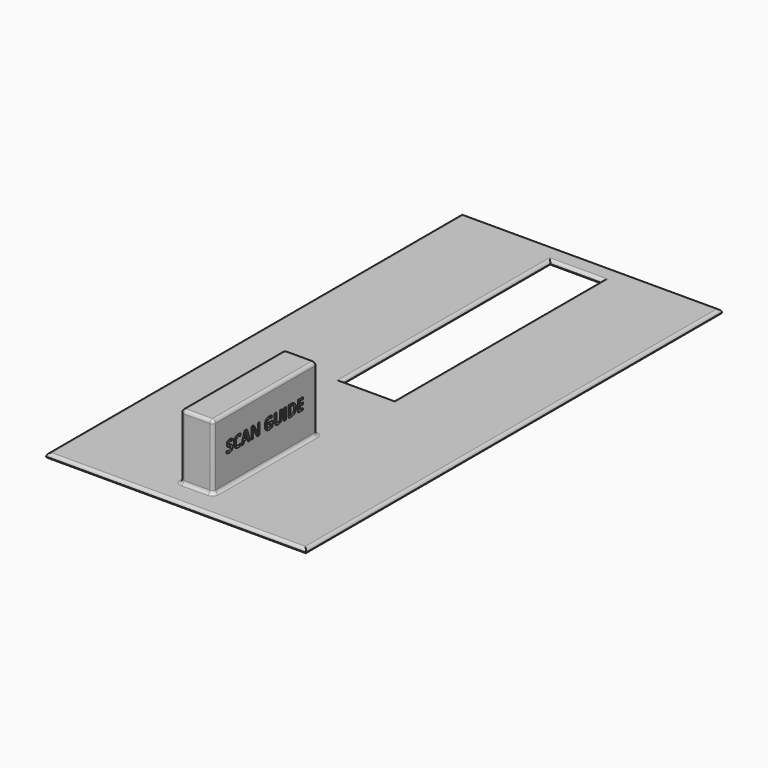
from build123d import *

# Parameters (mm, degrees)
F0_W          = 50.8
F0_H          = 101.5999981404
F1_DEPTH      = 1.016
F3_DEPTH      = 1.016
F4_DEPTH      = 12.7
F5_TEXT_SIZE  = 3.1394360757
F6_DEPTH      = 0.508
F7_TEXT_SIZE  = 2.617994417
F8_DEPTH      = 0.508
F9_R          = 0.635
F10_R         = 0.635
F11_T1_DEPTH  = 104.5099337067
F11_T3_DEPTH  = 53.7099355663
F11_T5_DEPTH  = 10.16
F11_T7_DEPTH  = 50.8
F11_T13_DEPTH = 11.6149677831
F11_T17_DEPTH = 52.2549677831
F11_T24_DEPTH = 52.2549677831
F11_T28_DEPTH = 11.6149677831
F11_T35_DEPTH = 52.2549677831
F11_T39_DEPTH = 11.6149677831
F11_T46_DEPTH = 11.6149677831
F11_T50_DEPTH = 52.2549677831


# Not quite as in the source:
# - a fillet or chamfer that OpenCascade refuses, or shapes differently, is made with other operations: its cross-section is extruded or revolved along the edge and cut away or added
# - Text() gives the source's letters only with a copy of the font that has no kerning and outlines rounded to 1/6400 em; it was checked with that copy


with BuildPart() as f1:
    # F0 (on Top) → F1 (new body)
    with BuildSketch(Plane.XY):
        with Locations((9.1255651787, -9.784890828)):
            Rectangle(F0_W, F0_H)
    extrude(amount=F1_DEPTH)

    # F2 (on face) → F3 (cut)
    with BuildSketch(Plane.XY.offset(1.016)):
        Polygon((4.0455651787, -13.5948917578), (9.1255651787, -13.5948917578), (14.2055651787, -13.5948917578), (14.2055651787, 37.2051082422), (9.1255651787, 37.2051082422), (4.0455651787, 37.2051082422), align=None)
    extrude(amount=-F3_DEPTH, mode=Mode.SUBTRACT)

    # F2 (on face) → F4 (join)
    with BuildSketch(Plane.XY.offset(1.016)):
        Polygon((12.3005651787, -30.1048898982), (9.1255651787, -30.1048898982), (5.9505651787, -30.1048898982), (5.9505651787, -55.5048898982), (9.1255651787, -55.5048898982), (12.3005651787, -55.5048898982), align=None)
    extrude(amount=F4_DEPTH)

    # F5 (on face) → F6 (cut)
    with BuildSketch(Plane.YZ.offset(12.3005651787)):
        with Locations((-52.3298898982, 6.7086623347)):
            Text('SCAN GUIDE', F5_TEXT_SIZE, font='Open Sans', font_style=FontStyle.BOLD, text_align=(TextAlign.LEFT, TextAlign.BOTTOM))
    extrude(amount=-F6_DEPTH, mode=Mode.SUBTRACT)

    # F7 (on face) → F8 (cut)
    with BuildSketch(Plane(origin=(5.9505651787, 0, 0), x_dir=(0, -1, 0), z_dir=(-1, 0, 0))):
        with Locations((33.1365615274, 6.3851709486)):
            Text('Physio Controls', F7_TEXT_SIZE, font='Open Sans', text_align=(TextAlign.LEFT, TextAlign.BOTTOM))
    extrude(amount=-F8_DEPTH, mode=Mode.SUBTRACT)

    # F9
    f9_edges = [f1.edges().sort_by_distance(p)[0] for p in [
        (12.300565, -42.80489, 1.016),
        (9.125565, -30.10489, 1.016),
        (5.950565, -42.80489, 1.016),
        (9.125565, -55.50489, 1.016),
        (9.125565, -30.10489, 13.716),
        (5.950565, -42.80489, 13.716),
        (9.125565, -55.50489, 13.716),
        (12.300565, -42.80489, 13.716),
        (5.950565, -55.50489, 7.366),
        (12.300565, -55.50489, 7.366),
        (12.300565, -30.10489, 7.366),
        (5.950565, -30.10489, 7.366),
    ]]
    fillet(f9_edges, radius=F9_R)

    # F10
    f10_edges = [f1.edges().sort_by_distance(p)[0] for p in [
        (12.935565, -42.80489, 1.016),
        (12.563591, -55.767916, 1.016),
        (12.563591, -29.841864, 1.016),
        (9.125565, -56.13989, 1.016),
        (9.125565, -29.46989, 1.016),
        (5.68754, -55.767916, 1.016),
        (5.68754, -29.841864, 1.016),
        (5.315565, -42.80489, 1.016),
        (34.525565, -9.784891, 1.016),
        (9.125565, -60.58489, 1.016),
        (9.125565, 41.015108, 1.016),
        (-16.274435, -9.784891, 1.016),
        (14.205565, 11.805108, 1.016),
        (9.125565, -13.594892, 1.016),
        (9.125565, 37.205108, 1.016),
        (4.045565, 11.805108, 1.016),
    ]]
    fillet(f10_edges, radius=F10_R)

    # F11: fillet of radius 0.635 on 8 edges, made by hand

    # F11_s2 → F11_t1 (cut)
    with BuildSketch(Plane.XZ.offset(-42.4700760253)):
        with BuildLine():
            ThreePointArc((34.5255651787, 0.381), (34.2913818894, 0.1037208832), (33.9435780654, 0))
            Line((33.9435780654, 0), (33.9435780654, -0.0127))
            Line((33.9435780654, -0.0127), (34.5255651787, -0.0127))
            Line((34.5255651787, -0.0127), (34.5382651787, 0))
            ThreePointArc((34.5382651787, 0), (34.5382651787, 0.1905), (34.537204921, 0.37592))
            Line((34.537204921, 0.37592), (34.5255651787, 0.381))
        make_face()
        with BuildLine():
            ThreePointArc((-16.2744348213, 0.381), (-16.0402515321, 0.1037208832), (-15.692447708, 0))
            Line((-15.692447708, 0), (-15.692447708, -0.0127))
            Line((-15.692447708, -0.0127), (-16.2744348213, -0.0127))
            Line((-16.2744348213, -0.0127), (-16.2871348213, 0))
            ThreePointArc((-16.2871348213, 0), (-16.2871348213, 0.1905), (-16.2860745636, 0.37592))
            Line((-16.2860745636, 0.37592), (-16.2744348213, 0.381))
        make_face()
    extrude(amount=F11_T1_DEPTH, mode=Mode.SUBTRACT)

    # F11_s4 → F11_t3 (cut)
    with BuildSketch(Plane.YZ.offset(-17.7294026045)):
        with BuildLine():
            ThreePointArc((-60.5848898982, 0.381), (-60.3507066089, 0.1037208832), (-60.0029027849, 0))
            Line((-60.0029027849, 0), (-60.0029027849, -0.0127))
            Line((-60.0029027849, -0.0127), (-60.5848898982, -0.0127))
            Line((-60.5848898982, -0.0127), (-60.5975898982, 0))
            ThreePointArc((-60.5975898982, 0), (-60.5975898982, 0.1905), (-60.5965296404, 0.37592))
            Line((-60.5965296404, 0.37592), (-60.5848898982, 0.381))
        make_face()
        with BuildLine():
            ThreePointArc((41.0151082422, 0.381), (40.7809249529, 0.1037208832), (40.4331211289, 0))
            Line((40.4331211289, 0), (40.4331211289, -0.0127))
            Line((40.4331211289, -0.0127), (41.0151082422, -0.0127))
            Line((41.0151082422, -0.0127), (41.0278082422, 0))
            ThreePointArc((41.0278082422, 0), (41.0278082422, 0.1905), (41.0267479844, 0.37592))
            Line((41.0267479844, 0.37592), (41.0151082422, 0.381))
        make_face()
    extrude(amount=F11_T3_DEPTH, mode=Mode.SUBTRACT)

    # F11_s6 → F11_t5 (cut)
    with BuildSketch(Plane.YZ.offset(4.0455651787)):
        with BuildLine():
            ThreePointArc((-13.5948917578, 0.381), (-13.8290750471, 0.1037208832), (-14.1768788711, 0))
            Line((-14.1768788711, 0), (-14.1768788711, -0.0127))
            Line((-14.1768788711, -0.0127), (-13.5948917578, -0.0127))
            Line((-13.5948917578, -0.0127), (-13.5821917578, 0))
            ThreePointArc((-13.5821917578, 0), (-13.5821917578, 0.1905), (-13.5832520156, 0.37592))
            Line((-13.5832520156, 0.37592), (-13.5948917578, 0.381))
        make_face()
        with BuildLine():
            ThreePointArc((37.2051082422, 0.381), (37.4392915314, 0.1037208832), (37.7870953554, 0))
            Line((37.7870953554, 0), (37.7870953554, -0.0127))
            Line((37.7870953554, -0.0127), (37.2051082422, -0.0127))
            Line((37.2051082422, -0.0127), (37.1924082422, 0))
            ThreePointArc((37.1924082422, 0), (37.1924082422, 0.1905), (37.1934684999, 0.37592))
            Line((37.1934684999, 0.37592), (37.2051082422, 0.381))
        make_face()
    extrude(amount=F11_T5_DEPTH, mode=Mode.SUBTRACT)

    # F11_s8 → F11_t7 (cut)
    with BuildSketch(Plane.XZ.offset(-37.2051082422)):
        with BuildLine():
            ThreePointArc((14.2055651787, 0.381), (14.4397484679, 0.1037208832), (14.787552292, 0))
            Line((14.787552292, 0), (14.787552292, -0.0127))
            Line((14.787552292, -0.0127), (14.2055651787, -0.0127))
            Line((14.2055651787, -0.0127), (14.1928651787, 0))
            ThreePointArc((14.1928651787, 0), (14.1928651787, 0.1905), (14.1939254364, 0.37592))
            Line((14.1939254364, 0.37592), (14.2055651787, 0.381))
        make_face()
        with BuildLine():
            ThreePointArc((4.0455651787, 0.381), (3.8113818894, 0.1037208832), (3.4635780654, 0))
            Line((3.4635780654, 0), (3.4635780654, -0.0127))
            Line((3.4635780654, -0.0127), (4.0455651787, -0.0127))
            Line((4.0455651787, -0.0127), (4.0582651787, 0))
            ThreePointArc((4.0582651787, 0), (4.0582651787, 0.1905), (4.057204921, 0.37592))
            Line((4.057204921, 0.37592), (4.0455651787, 0.381))
        make_face()
    extrude(amount=F11_T7_DEPTH, mode=Mode.SUBTRACT)


with BuildPart() as f11_tool11:
    # F11_s12 → F11_t13 (new body)
    with BuildSketch(Plane.YZ.offset(2.5905973955)):
        with BuildLine():
            ThreePointArc((-13.5948917578, 0.381), (-13.8290750471, 0.1037208832), (-14.1768788711, 0))
            Line((-14.1768788711, 0), (-14.1768788711, -0.0127))
            Line((-14.1768788711, -0.0127), (-13.5948917578, -0.0127))
            Line((-13.5948917578, -0.0127), (-13.5821917578, 0))
            ThreePointArc((-13.5821917578, 0), (-13.5821917578, 0.1905), (-13.5832520156, 0.37592))
            Line((-13.5832520156, 0.37592), (-13.5948917578, 0.381))
        make_face()
    extrude(amount=F11_T13_DEPTH)

    split(bisect_by=Plane.YZ.offset(4.0455651787), keep=Keep.BOTTOM)


with BuildPart() as f11_tool15:
    # F11_s16 → F11_t17 (new body)
    with BuildSketch(Plane.XZ.offset(-37.2051082422)):
        with BuildLine():
            ThreePointArc((4.0455651787, 0.381), (3.8113818894, 0.1037208832), (3.4635780654, 0))
            Line((3.4635780654, 0), (3.4635780654, -0.0127))
            Line((3.4635780654, -0.0127), (4.0455651787, -0.0127))
            Line((4.0455651787, -0.0127), (4.0582651787, 0))
            ThreePointArc((4.0582651787, 0), (4.0582651787, 0.1905), (4.057204921, 0.37592))
            Line((4.057204921, 0.37592), (4.0455651787, 0.381))
        make_face()
    extrude(amount=F11_T17_DEPTH)

    split(bisect_by=Plane.XZ.offset(13.5948917578), keep=Keep.TOP)


with BuildPart() as f11_tool11_1:
    add(f11_tool11.part)

    # F11_t19: intersect F11_tool15
    add(f11_tool15.part, mode=Mode.INTERSECT)


with BuildPart() as f1_1:
    add(f1.part)

    # F11_t9: cut F11_tool11
    add(f11_tool11_1.part, mode=Mode.SUBTRACT)


with BuildPart() as f11_tool22:
    # F11_s23 → F11_t24 (new body)
    with BuildSketch(Plane.XZ.offset(15.049859541)):
        with BuildLine():
            ThreePointArc((14.2055651787, 0.381), (14.4397484679, 0.1037208832), (14.787552292, 0))
            Line((14.787552292, 0), (14.787552292, -0.0127))
            Line((14.787552292, -0.0127), (14.2055651787, -0.0127))
            Line((14.2055651787, -0.0127), (14.1928651787, 0))
            ThreePointArc((14.1928651787, 0), (14.1928651787, 0.1905), (14.1939254364, 0.37592))
            Line((14.1939254364, 0.37592), (14.2055651787, 0.381))
        make_face()
    extrude(amount=-F11_T24_DEPTH)

    split(bisect_by=Plane.XZ.offset(13.5948917578), keep=Keep.TOP)


with BuildPart() as f11_tool26:
    # F11_s27 → F11_t28 (new body)
    with BuildSketch(Plane.YZ.offset(4.0455651787)):
        with BuildLine():
            ThreePointArc((-13.5948917578, 0.381), (-13.8290750471, 0.1037208832), (-14.1768788711, 0))
            Line((-14.1768788711, 0), (-14.1768788711, -0.0127))
            Line((-14.1768788711, -0.0127), (-13.5948917578, -0.0127))
            Line((-13.5948917578, -0.0127), (-13.5821917578, 0))
            ThreePointArc((-13.5821917578, 0), (-13.5821917578, 0.1905), (-13.5832520156, 0.37592))
            Line((-13.5832520156, 0.37592), (-13.5948917578, 0.381))
        make_face()
    extrude(amount=F11_T28_DEPTH)

    split(bisect_by=Plane.YZ.offset(14.2055651787), keep=Keep.TOP)


with BuildPart() as f11_tool22_1:
    add(f11_tool22.part)

    # F11_t30: intersect F11_tool26
    add(f11_tool26.part, mode=Mode.INTERSECT)


with BuildPart() as f1_2:
    add(f1_1.part)

    # F11_t20: cut F11_tool22
    add(f11_tool22_1.part, mode=Mode.SUBTRACT)


with BuildPart() as f11_tool33:
    # F11_s34 → F11_t35 (new body)
    with BuildSketch(Plane.XZ.offset(13.5948917578)):
        with BuildLine():
            ThreePointArc((14.2055651787, 0.381), (14.4397484679, 0.1037208832), (14.787552292, 0))
            Line((14.787552292, 0), (14.787552292, -0.0127))
            Line((14.787552292, -0.0127), (14.2055651787, -0.0127))
            Line((14.2055651787, -0.0127), (14.1928651787, 0))
            ThreePointArc((14.1928651787, 0), (14.1928651787, 0.1905), (14.1939254364, 0.37592))
            Line((14.1939254364, 0.37592), (14.2055651787, 0.381))
        make_face()
    extrude(amount=-F11_T35_DEPTH)

    split(bisect_by=Plane.XZ.offset(-37.2051082422), keep=Keep.BOTTOM)


with BuildPart() as f11_tool37:
    # F11_s38 → F11_t39 (new body)
    with BuildSketch(Plane.YZ.offset(15.6605329618)):
        with BuildLine():
            ThreePointArc((37.2051082422, 0.381), (37.4392915314, 0.1037208832), (37.7870953554, 0))
            Line((37.7870953554, 0), (37.7870953554, -0.0127))
            Line((37.7870953554, -0.0127), (37.2051082422, -0.0127))
            Line((37.2051082422, -0.0127), (37.1924082422, 0))
            ThreePointArc((37.1924082422, 0), (37.1924082422, 0.1905), (37.1934684999, 0.37592))
            Line((37.1934684999, 0.37592), (37.2051082422, 0.381))
        make_face()
    extrude(amount=-F11_T39_DEPTH)

    split(bisect_by=Plane.YZ.offset(14.2055651787), keep=Keep.TOP)


with BuildPart() as f11_tool33_1:
    add(f11_tool33.part)

    # F11_t41: intersect F11_tool37
    add(f11_tool37.part, mode=Mode.INTERSECT)


with BuildPart() as f1_3:
    add(f1_2.part)

    # F11_t31: cut F11_tool33
    add(f11_tool33_1.part, mode=Mode.SUBTRACT)


with BuildPart() as f11_tool44:
    # F11_s45 → F11_t46 (new body)
    with BuildSketch(Plane.YZ.offset(14.2055651787)):
        with BuildLine():
            ThreePointArc((37.2051082422, 0.381), (37.4392915314, 0.1037208832), (37.7870953554, 0))
            Line((37.7870953554, 0), (37.7870953554, -0.0127))
            Line((37.7870953554, -0.0127), (37.2051082422, -0.0127))
            Line((37.2051082422, -0.0127), (37.1924082422, 0))
            ThreePointArc((37.1924082422, 0), (37.1924082422, 0.1905), (37.1934684999, 0.37592))
            Line((37.1934684999, 0.37592), (37.2051082422, 0.381))
        make_face()
    extrude(amount=-F11_T46_DEPTH)

    split(bisect_by=Plane.YZ.offset(4.0455651787), keep=Keep.BOTTOM)


with BuildPart() as f11_tool48:
    # F11_s49 → F11_t50 (new body)
    with BuildSketch(Plane.XZ.offset(-38.6600760253)):
        with BuildLine():
            ThreePointArc((4.0455651787, 0.381), (3.8113818894, 0.1037208832), (3.4635780654, 0))
            Line((3.4635780654, 0), (3.4635780654, -0.0127))
            Line((3.4635780654, -0.0127), (4.0455651787, -0.0127))
            Line((4.0455651787, -0.0127), (4.0582651787, 0))
            ThreePointArc((4.0582651787, 0), (4.0582651787, 0.1905), (4.057204921, 0.37592))
            Line((4.057204921, 0.37592), (4.0455651787, 0.381))
        make_face()
    extrude(amount=F11_T50_DEPTH)

    split(bisect_by=Plane.XZ.offset(-37.2051082422), keep=Keep.BOTTOM)


with BuildPart() as f11_tool44_1:
    add(f11_tool44.part)

    # F11_t52: intersect F11_tool48
    add(f11_tool48.part, mode=Mode.INTERSECT)


with BuildPart() as f1_4:
    add(f1_3.part)

    # F11_t42: cut F11_tool44
    add(f11_tool44_1.part, mode=Mode.SUBTRACT)


solid = f1_4.part
